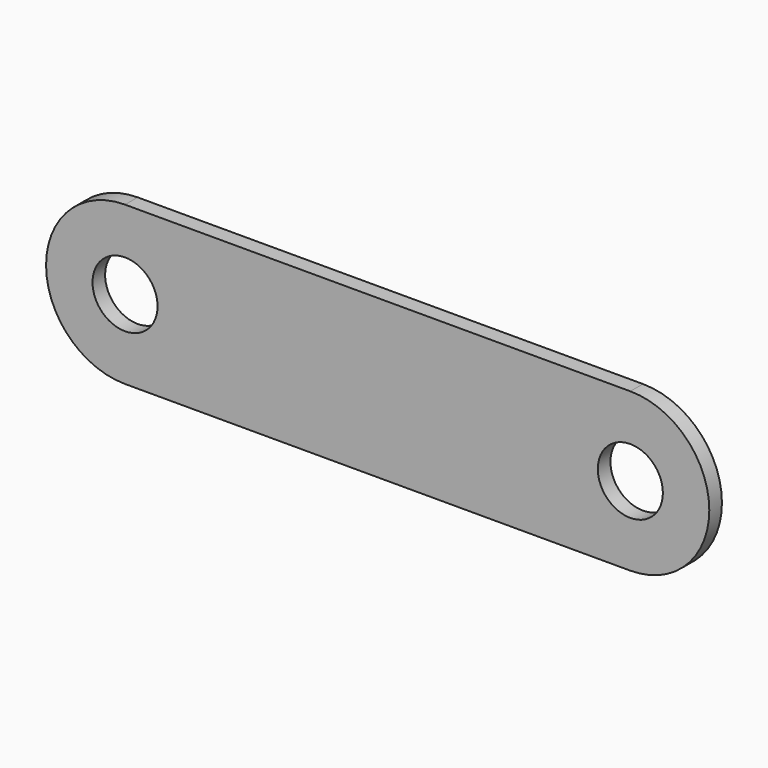
from build123d import *

# Parameters (mm, degrees)
F0_R     = 6.5405
F1_DEPTH = 1.5875


# Not quite as in the source:
# - a length typed as a fraction of an inch, garbled in the dataset ("3 / 203.2 mm" for 3/8 in), is restored


with BuildPart() as f1:
    # F0 (on Front) → F1 (new body, symmetric)
    with BuildSketch(Plane.XZ):
        with BuildLine():
            Line((0, 15.875), (-50.8, 15.875))
            ThreePointArc((-50.8, 15.875), (-66.675, 0), (-50.8, -15.875))
            Line((-50.8, -15.875), (0, -15.875))
            Line((0, -15.875), (50.8, -15.875))
            ThreePointArc((50.8, -15.875), (66.675, 0), (50.8, 15.875))
            Line((50.8, 15.875), (0, 15.875))
        make_face()
        with Locations((-50.8, 0)):
            Circle(F0_R, mode=Mode.SUBTRACT)
        with Locations((50.8, 0)):
            Circle(F0_R, mode=Mode.SUBTRACT)
    extrude(amount=F1_DEPTH, both=True)


solid = f1.part
